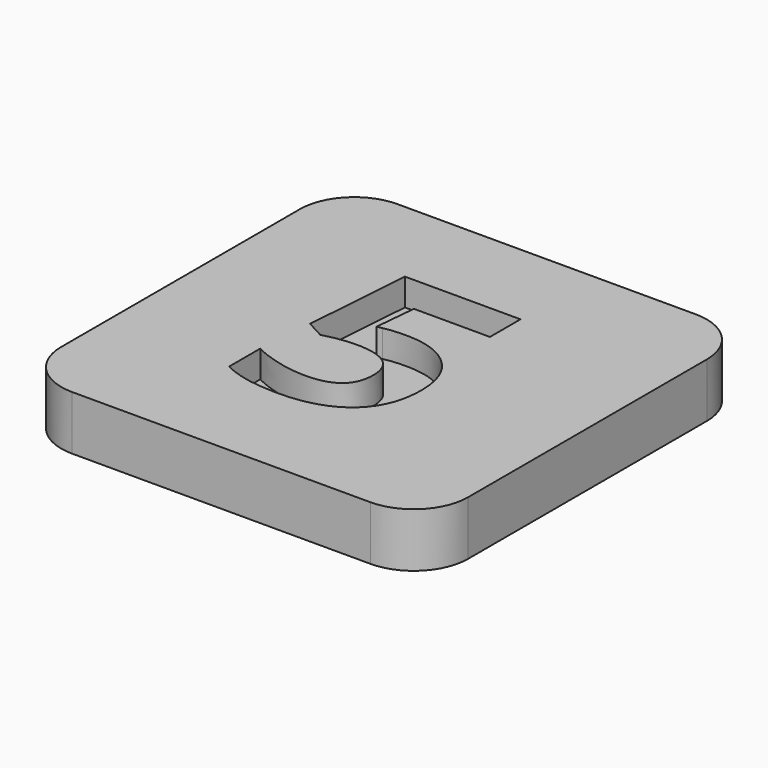
from build123d import *

# Parameters (mm, degrees)
F0_W         = 38.1
F0_H         = 38.1
F1_DEPTH     = 5.08
F2_TEXT_SIZE = 27.9460460196
F3_DEPTH     = 2.54
F4_R         = 5.08


# Not quite as in the source:
# - Text() gives the source's letters only with a copy of the font that has no kerning and outlines rounded to 1/6400 em; it was checked with that copy


with BuildPart() as f1:
    # F0 (on Top) → F1 (new body)
    with BuildSketch(Plane.XY):
        Rectangle(F0_W, F0_H)
    extrude(amount=F1_DEPTH)

    # F2 (on face) → F3 (cut)
    with BuildSketch(Plane.XY.offset(5.08)):
        with Locations((-8.89, -9.525)):
            Text('5', F2_TEXT_SIZE, font='Open Sans', font_style=FontStyle.BOLD, text_align=(TextAlign.LEFT, TextAlign.BOTTOM))
    extrude(amount=-F3_DEPTH, mode=Mode.SUBTRACT)

    # F4
    f4_edges = [f1.edges().sort_by_distance(p)[0] for p in [
        (-19.05, -19.05, 2.54),
        (19.05, -19.05, 2.54),
        (19.05, 19.05, 2.54),
        (-19.05, 19.05, 2.54),
    ]]
    fillet(f4_edges, radius=F4_R)


solid = f1.part
